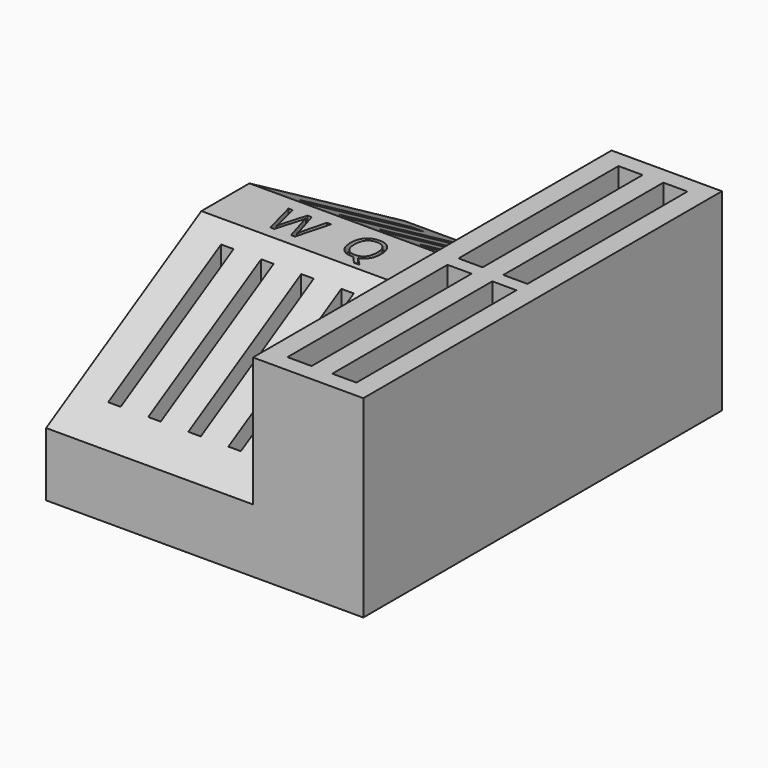
from build123d import *

# Parameters (mm, degrees)
F0_W           = 58.42
F0_H           = 82.55
F1_DEPTH       = 35.56
F2_W           = 2.3
F2_H           = 26
F3_DEPTH       = 31.75
F5_DEPTH       = 38.1
F6_W           = 4.445
F6_H           = 36.83
F7_DEPTH       = 31.75
F8_TEXT_SIZE   = 8.7376509327
F8_TEXT_SIZE_2 = 8.5989579222
F9_DEPTH       = 1.27


# Not quite as in the source:
# - Text() gives the source's letters only with a copy of the font that has no kerning and outlines rounded to 1/6400 em; it was checked with that copy


with BuildPart() as f1:
    # F0 (on Top) → F1 (new body)
    with BuildSketch(Plane.XY):
        Rectangle(F0_W, F0_H)
    extrude(amount=F1_DEPTH)

    # F2 (on face) → F3 (cut)
    with BuildSketch(Plane.XY.offset(35.56)):
        with Locations((-21.71, 21.925)):
            Rectangle(F2_W, F2_H)
        with Locations((-14.33, 21.925)):
            Rectangle(F2_W, F2_H)
        with Locations((-6.95, 21.925)):
            Rectangle(F2_W, F2_H)
        with Locations((0.43, 21.925)):
            Rectangle(F2_W, F2_H)
        with Locations((0.43, -21.925)):
            Rectangle(F2_W, F2_H)
        with Locations((-6.95, -21.925)):
            Rectangle(F2_W, F2_H)
        with Locations((-14.33, -21.925)):
            Rectangle(F2_W, F2_H)
        with Locations((-21.71, -21.925)):
            Rectangle(F2_W, F2_H)
    extrude(amount=-F3_DEPTH, mode=Mode.SUBTRACT)

    # F4 (on face) → F5 (cut)
    with BuildSketch(Plane(origin=(-29.21, 0, 0), x_dir=(0, -1, 0), z_dir=(-1, 0, 0))):
        Polygon((-5.5253629041, 32.3699302399), (0, 35.56), (-41.275, 35.56), (-41.275, 11.7298676392), align=None)
        Polygon((41.275, 35.56), (0, 35.56), (5.5253629041, 32.3699302399), (41.275, 11.7298676392), align=None)
        Polygon((5.5253629041, 32.3699302399), (0, 35.56), (-5.5253629041, 32.3699302399), align=None)
    extrude(amount=-F5_DEPTH, mode=Mode.SUBTRACT)

    # F6 (on face) → F7 (cut)
    with BuildSketch(Plane.XY.offset(35.56)):
        with Locations((14.9225, 19.685)):
            Rectangle(F6_W, F6_H)
        with Locations((23.1775, 19.685)):
            Rectangle(F6_W, F6_H)
        with Locations((14.9225, -19.685)):
            Rectangle(F6_W, F6_H)
        with Locations((23.1775, -19.685)):
            Rectangle(F6_W, F6_H)
    extrude(amount=-F7_DEPTH, mode=Mode.SUBTRACT)

    # F8 (on face) → F9 (cut)
    with BuildSketch(Plane.XY.offset(32.3699302399)):
        with Locations((-20.0417684391, -3.3285535901)):
            Text('W', F8_TEXT_SIZE, font='Open Sans', text_align=(TextAlign.LEFT, TextAlign.BOTTOM))
        with Locations((-6.8166735582, -2.9281987809)):
            Text('Q', F8_TEXT_SIZE_2, font='Open Sans', text_align=(TextAlign.LEFT, TextAlign.BOTTOM))
    extrude(amount=-F9_DEPTH, mode=Mode.SUBTRACT)


solid = f1.part
